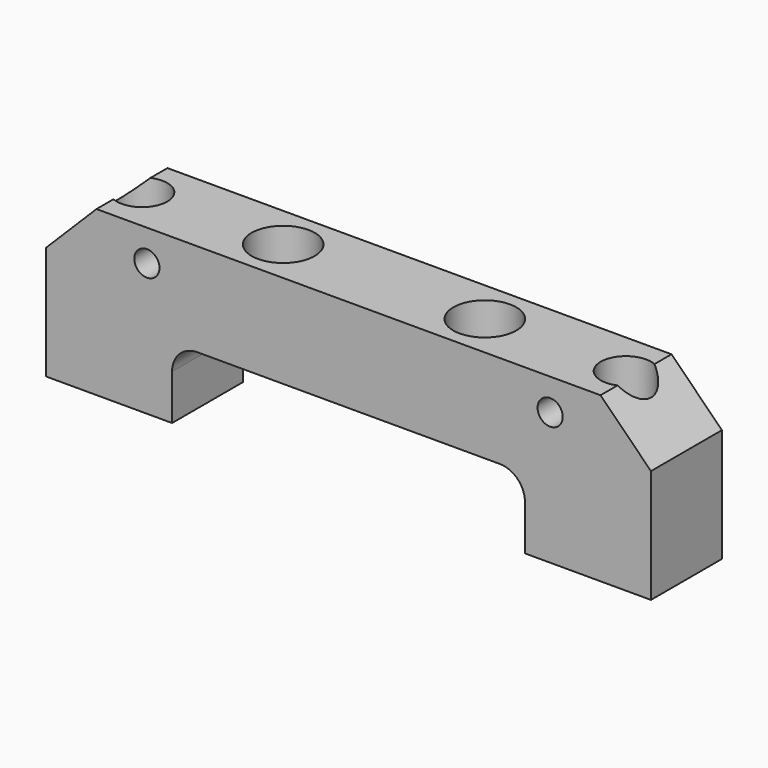
from build123d import *

# Parameters (mm, degrees)
F1_DEPTH       = 11.176
F2_R           = 3.175
F5_D           = 3.4544
F5_START       = 10.33145
F5_CBORE_D     = 6.35
F5_CBORE_DEPTH = 11.7602
F6_T1_DEPTH    = 43.8363739472
F8_D           = 7.9375
F10_D          = 3.175


# Not quite as in the source:
# - a fillet or chamfer that OpenCascade refuses, or shapes differently, is made with other operations: its cross-section is extruded or revolved along the edge and cut away or added


with BuildPart() as f1:
    # F0 (on Front) → F1 (new body)
    with BuildSketch(Plane.XZ):
        Polygon((38.1, 10.31875), (-38.1, 10.31875), (-38.1, -10.31875), (-22.225, -10.31875), (-22.225, -1.42875), (22.225, -1.42875), (22.225, -10.31875), (38.1, -10.31875), align=None)
    extrude(amount=F1_DEPTH)

    # F2
    f2_edges = [f1.edges().sort_by_distance(p)[0] for p in [
        (-22.225, -5.588, -1.42875),
        (22.225, -5.588, -1.42875),
    ]]
    fillet(f2_edges, radius=F2_R)

    # F5 (through all)
    # its depths count from where the whole tool has entered the part; down to there all is cleared
    with Locations(Plane.XY.offset(20.6502).offset(-F5_START)):
        with Locations((-30.48, -5.588), (30.48, -5.588)):
            CounterBoreHole(F5_D / 2, F5_CBORE_D / 2, F5_CBORE_DEPTH)

    # F6: chamfer of 6.35 on 2 edges, made by hand

    # F6_s2 → F6_t1 (cut)
    with BuildSketch(Plane.XZ.offset(-16.3301869736)):
        Polygon((-38.1, 3.96875), (-31.75, 10.31875), (-38.1, 10.31875), align=None)
        Polygon((31.75, 10.31875), (38.1, 3.96875), (38.1, 10.31875), align=None)
    extrude(amount=F6_T1_DEPTH, mode=Mode.SUBTRACT)

    # F8 (through all)
    with Locations(Plane.XY.offset(20.6502)):
        with Locations((-12.7, -5.588), (12.7, -5.588)):
            Hole(F8_D / 2)

    # F10 (through all)
    with Locations(Plane.XZ.offset(11.176)):
        with Locations((-25.4, 6.35635), (25.4, 6.35635)):
            Hole(F10_D / 2)


solid = f1.part
